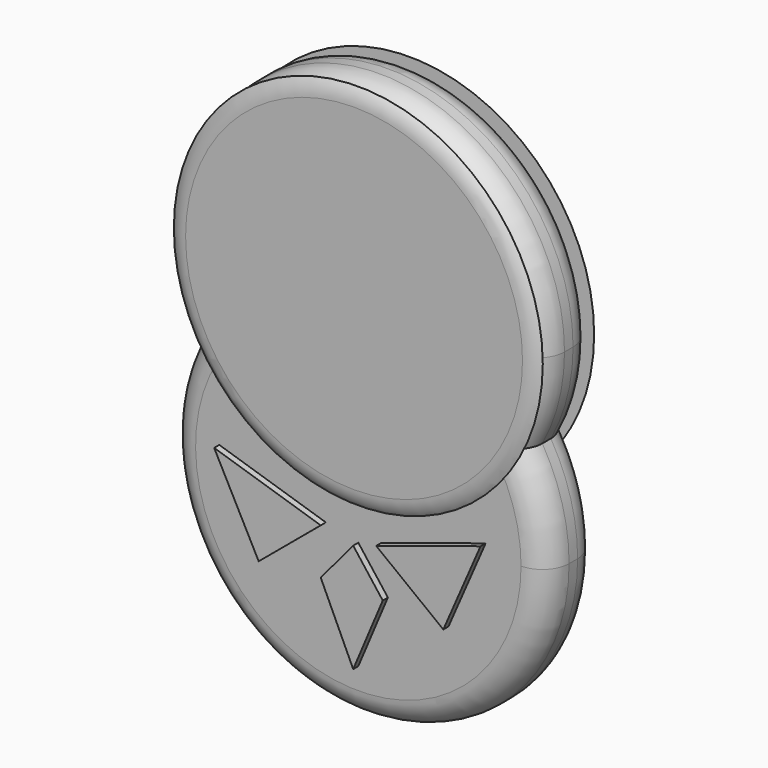
from build123d import *

# Parameters (mm, degrees)
F2_DEPTH  = 12
F3_R      = 34.5596159482
F4_DEPTH  = 1
F5_R      = 34.5816890446
F6_DEPTH  = 1
F7_F1_R   = 5
F10_DEPTH = 1.2


# Not quite as in the source:
# - a fillet or chamfer that OpenCascade refuses, or shapes differently, is made with other operations: its cross-section is extruded or revolved along the edge and cut away or added


with BuildPart() as f2:
    # F0 (on Front) → F2 (new body)
    with BuildSketch(Plane.XZ):
        with BuildLine():
            ThreePointArc((30.4762787484, 9.9597305745), (33.5754539102, 17.9238433098), (34.6299175574, 26.404414326))
            ThreePointArc((34.6299175574, 26.404414326), (-8.4805710162, 59.9798682361), (-30.4762787484, 9.9597305745))
            ThreePointArc((-30.4762787484, 9.9597305745), (0, 27.2640205034), (30.4762787484, 9.9597305745))
        make_face()
        with BuildLine():
            ThreePointArc((30.4762787484, 9.9597305745), (0, 27.2640205034), (-30.4762787484, 9.9597305745))
            ThreePointArc((-30.4762787484, 9.9597305745), (0, -8.2255032315), (30.4762787484, 9.9597305745))
        make_face()
        with BuildLine():
            ThreePointArc((30.4762787484, 9.9597305745), (0, -8.2255032315), (-30.4762787484, 9.9597305745))
            ThreePointArc((-30.4762787484, 9.9597305745), (-9.431799323, -42.4387675666), (35.4895237349, -8.2255032315))
            ThreePointArc((35.4895237349, -8.2255032315), (34.2132643351, 1.2062960915), (30.4762787484, 9.9597305745))
        make_face()
    extrude(amount=F2_DEPTH)

    # F7: fillet of radius 5 on 4 edges, made by hand

    # F7_f1
    f7_f1_edges = [f2.edges().sort_by_distance(p)[0] for p in [
        (0, -12, -43.7150269664),
        (0, -12, 61.0343318834),
        (0, 0, -43.7150269664),
        (0, 0, 61.0343318834),
    ]]
    fillet(f7_f1_edges, radius=F7_F1_R)

    # F9 (on face) → F10 (join)
    with BuildSketch(Plane.XZ.offset(12)):
        Polygon((-6.0839848593, -12.9199223593), (-26.0449238122, -6.6308598034), (-17.7050791681, -22.6269550622), align=None)
        Polygon((23.857422173, -6.6308598034), (4.306640476, -12.9199223593), (16.8847665191, -22.6269550622), align=None)
        Polygon((5.5371099152, -21.5332042426), (0, -14.2871094868), (-6.0839848593, -21.5332042426), (0, -34.6582047641), align=None)
    extrude(amount=F10_DEPTH)


with BuildPart() as f4:
    # F3 (on face) → F4 (new body)
    with BuildSketch(Plane.XZ.offset(12)):
        with Locations((0, 26.404414326)):
            Circle(F3_R)
    extrude(amount=F4_DEPTH)

    # F8: fillet of radius 5 on 1 edges, made by hand

    # F8_s1 → F8_t2 (revolve, cut)
    with BuildSketch(Plane.XY.offset(26.404414326)):
        with BuildLine():
            ThreePointArc((34.5596159482, -12), (33.1407547783, -12.7434164903), (31.5596159482, -13))
            Line((31.5596159482, -13), (34.5596159482, -13))
            Line((34.5596159482, -13), (34.5596159482, -12))
        make_face()
    revolve(axis=Axis((0, -13, 26.404414326), (0, -1, 0)), mode=Mode.SUBTRACT)


with BuildPart() as f6:
    # F5 (on face) → F6 (new body)
    with BuildSketch(Plane(origin=(0, 0, 0), x_dir=(-1, 0, 0), z_dir=(0, 1, 0))):
        with Locations((0, 26.404414326)):
            Circle(F5_R)
    extrude(amount=F6_DEPTH)

    # F7#2: fillet of radius 5 on 1 edges, made by hand

    # F7_2_s1 → F7_2_t2 (revolve, cut)
    with BuildSketch(Plane.XY.offset(26.404414326)):
        with BuildLine():
            ThreePointArc((-34.5816890446, 0), (-33.1628278747, 0.7434164903), (-31.5816890446, 1))
            Line((-31.5816890446, 1), (-34.5816890446, 1))
            Line((-34.5816890446, 1), (-34.5816890446, 0))
        make_face()
    revolve(axis=Axis((0, 1, 26.404414326), (0, 1, 0)), mode=Mode.SUBTRACT)


solid = Compound([f2.part, f4.part, f6.part])
